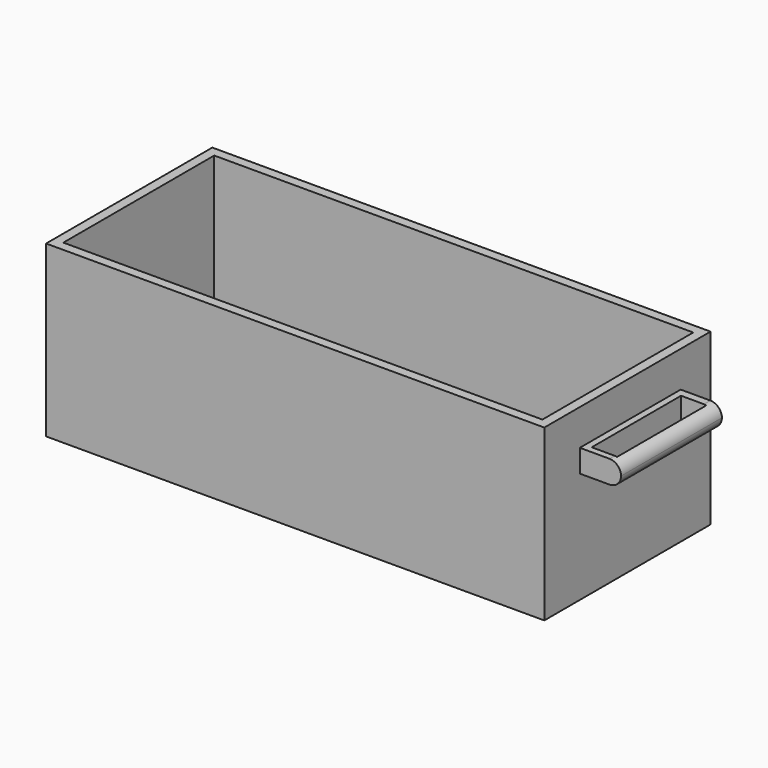
from build123d import *

# Parameters (mm, degrees)
F0_W         = 131.8914890289
F0_H         = 55.0068765879
F1_DEPTH     = 44.958
F2_T         = -2.54
F3_W         = 33.3715188317
F3_H         = 6.021162495
F4_DEPTH     = 10.922
F5_W         = 6.7100599408
F5_H         = 29.552442953
F6_DEPTH     = 25.4
F7_T1_DEPTH  = 48.7017749528
F8_W         = 30.4629029706
F8_H         = 4.9823708832
F9_DEPTH     = 8.128
F10_W        = 5.0006210804
F10_H        = 27.0441961475
F11_DEPTH    = 25.4
F12_T1_DEPTH = 45.7931590917


# Not quite as in the source:
# - a fillet or chamfer that OpenCascade refuses, or shapes differently, is made with other operations: its cross-section is extruded or revolved along the edge and cut away or added


with BuildPart() as f1:
    # F0 (on Top) → F1 (new body)
    with BuildSketch(Plane.XY):
        with Locations((0.1562684774, 11.095136404)):
            Rectangle(F0_W, F0_H)
    extrude(amount=F1_DEPTH)

    # F2
    f2_openings = [f1.faces().sort_by_distance(p)[0] for p in [
        (0.156268, 11.095136, 44.958),
    ]]
    offset(amount=F2_T, openings=f2_openings)

    # F3 (on face) → F4 (join)
    with BuildSketch(Plane.YZ.offset(66.1020129919)):
        with Locations((12.0295642409, 32.4530350044)):
            Rectangle(F3_W, F3_H)
    extrude(amount=F4_DEPTH)

    # F5 (on face) → F6 (cut)
    with BuildSketch(Plane.XY.offset(35.4636162519)):
        with Locations((71.2361820042, 11.8320556358)):
            Rectangle(F5_W, F5_H)
    extrude(amount=-F6_DEPTH, mode=Mode.SUBTRACT)

    # F7: fillet of radius 3.0660512242 on 2 edges, made by hand

    # F7_s2 → F7_t1 (cut)
    with BuildSketch(Plane.XZ.offset(-36.3804517173)):
        with BuildLine():
            ThreePointArc((73.9579617677, 35.4636162519), (76.1259873798, 34.5655906398), (77.0240129919, 32.3975650277))
            Line((77.0240129919, 32.3975650277), (77.0240129919, 35.4636162519))
            Line((77.0240129919, 35.4636162519), (73.9579617677, 35.4636162519))
        make_face()
        with BuildLine():
            ThreePointArc((73.9579617677, 29.4424537569), (76.1259873798, 30.340479369), (77.0240129919, 32.5085049811))
            Line((77.0240129919, 32.5085049811), (77.0240129919, 29.4424537569))
            Line((77.0240129919, 29.4424537569), (73.9579617677, 29.4424537569))
        make_face()
    extrude(amount=F7_T1_DEPTH, mode=Mode.SUBTRACT)

    # F8 (on face) → F9 (join)
    with BuildSketch(Plane(origin=(-65.789476037, 0, 0), x_dir=(0, -1, 0), z_dir=(-1, 0, 0))):
        with Locations((-11.8714510463, 30.9710260481)):
            Rectangle(F8_W, F8_H)
    extrude(amount=F9_DEPTH)

    # F10 (on face) → F11 (cut)
    with BuildSketch(Plane.XY.offset(33.4622114897)):
        with Locations((-69.5076957345, 11.8382142391)):
            Rectangle(F10_W, F10_H)
    extrude(amount=-F11_DEPTH, mode=Mode.SUBTRACT)

    # F12: fillet of radius 3.0660512242 on 2 edges, made by hand

    # F12_s2 → F12_t1 (cut)
    with BuildSketch(Plane.XZ.offset(-34.7680305922)):
        with BuildLine():
            ThreePointArc((-70.8514248128, 33.4622114897), (-73.0194504249, 32.5641858776), (-73.917476037, 30.3961602655))
            Line((-73.917476037, 30.3961602655), (-73.917476037, 33.4622114897))
            Line((-73.917476037, 33.4622114897), (-70.8514248128, 33.4622114897))
        make_face()
        with BuildLine():
            ThreePointArc((-70.8514248128, 28.4798406065), (-73.0194504249, 29.3778662186), (-73.917476037, 31.5458918307))
            Line((-73.917476037, 31.5458918307), (-73.917476037, 28.4798406065))
            Line((-73.917476037, 28.4798406065), (-70.8514248128, 28.4798406065))
        make_face()
    extrude(amount=F12_T1_DEPTH, mode=Mode.SUBTRACT)


solid = f1.part
